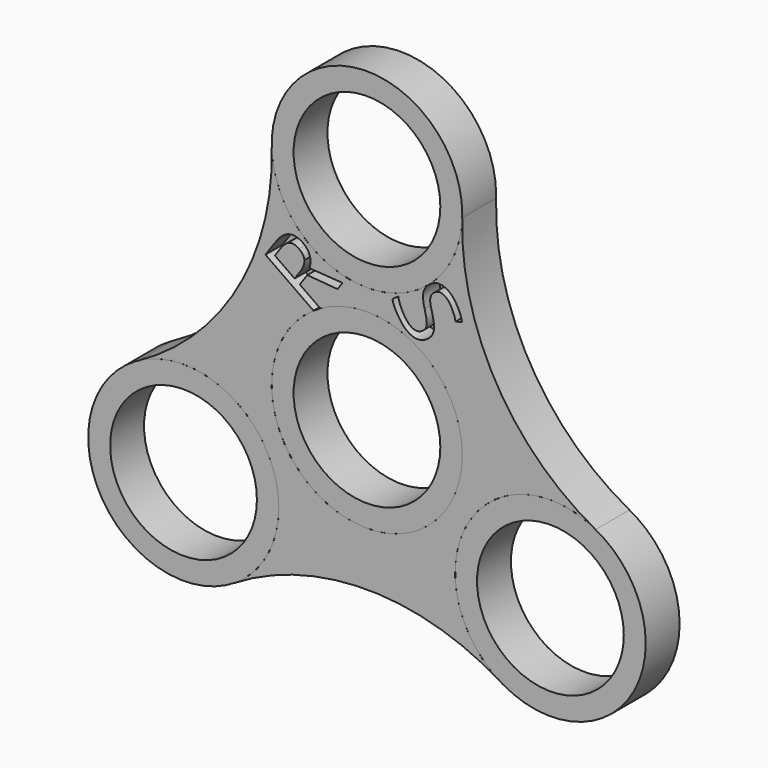
from build123d import *

# Parameters (mm, degrees)
F0_R         = 14.2875
F0_R_2       = 10.9982
F2_DEPTH     = 6.35
F1_R         = 14.2875
F3_TEXT_SIZE = 13.2291666667
F4_DEPTH     = 3.175


# Not quite as in the source:
# - Text() gives the source's letters only with a copy of the font that has no kerning and outlines rounded to 1/6400 em; it was checked with that copy


with BuildPart() as f2:
    # F0 (on Front) → F2 (new body)
    with BuildSketch(Plane.XZ):
        with Locations((0, 31.75)):
            Circle(F0_R)
        with Locations((0, 31.75)):
            Circle(F0_R_2, mode=Mode.SUBTRACT)
    extrude(amount=F2_DEPTH)


with BuildPart() as f2b:
    # F0 (on Front) → F2, piece 2 (new body)
    with BuildSketch(Plane.XZ):
        with Locations((-27.4963065702, -15.875)):
            Circle(F0_R)
        with Locations((-27.4963065702, -15.875)):
            Circle(F0_R_2, mode=Mode.SUBTRACT)
    extrude(amount=F2_DEPTH)


with BuildPart() as f2c:
    # F0 (on Front) → F2, piece 3 (new body)
    with BuildSketch(Plane.XZ):
        Circle(F0_R)
        Circle(F0_R_2, mode=Mode.SUBTRACT)
    extrude(amount=F2_DEPTH)


with BuildPart() as f2d:
    # F0 (on Front) → F2, piece 4 (new body)
    with BuildSketch(Plane.XZ):
        with Locations((27.4963065702, -15.875)):
            Circle(F0_R)
        with Locations((27.4963065702, -15.875)):
            Circle(F0_R_2, mode=Mode.SUBTRACT)
    extrude(amount=F2_DEPTH)


with BuildPart() as f2e:
    # F1 (on face) → F2, piece 5 (new body)
    with BuildSketch(Plane.XZ):
        with BuildLine():
            ThreePointArc((14.281510571, 31.3363430635), (0, 17.4625), (-14.281510571, 31.3363430635))
            ThreePointArc((-14.281510571, 31.3363430635), (-19.3699708761, 11.1832578995), (-34.2788244402, -3.3000205729))
            ThreePointArc((-34.2788244402, -3.3000205729), (-20.1741678054, -3.6063839346), (-13.2088065702, -15.875))
            ThreePointArc((-13.2088065702, -15.875), (-15.0208403571, -22.8388637995), (-19.9973138692, -28.0363224906))
            ThreePointArc((-19.9973138692, -28.0363224906), (0, -22.366515799), (19.9973138692, -28.0363224906))
            ThreePointArc((19.9973138692, -28.0363224906), (15.1229686136, -8.73125), (34.2788244402, -3.3000205729))
            ThreePointArc((34.2788244402, -3.3000205729), (19.3699708761, 11.1832578995), (14.281510571, 31.3363430635))
        make_face()
        Circle(F1_R, mode=Mode.SUBTRACT)
    extrude(amount=F2_DEPTH)

    # F3 (on face) → F4 (cut)
    with BuildSketch(Plane.XZ.offset(6.35)):
        with BuildLine():
            Line((-6.9997403161, 12.4553720039), (-10.0711094385, 14.605967816))
            Line((-10.0711094385, 14.605967816), (-8.9400323897, 16.2213132487))
            Line((-8.9400323897, 16.2213132487), (-4.4115968154, 15.841361106))
            Line((-4.4115968154, 15.841361106), (-3.6670303724, 16.9047121874))
            Line((-3.6670303724, 16.9047121874), (-8.6145888532, 17.2374768616))
            add(Edge.make_bspline(
                [(-9.5992202444, 20.245937907), (-8.0651500536, 19.1717703953), (-8.6145888532, 17.2374768616)],
                knots=[0, 0, 0, 1, 1, 1], degree=2))
            add(Edge.make_bspline(
                [(-11.7159887552, 20.7149656524), (-10.6947427758, 21.0130310418), (-9.5992202444, 20.245937907)],
                knots=[0, 0, 0, 1, 1, 1], degree=2))
            add(Edge.make_bspline(
                [(-13.7343372483, 18.9928902956), (-12.7372347346, 20.4169002629), (-11.7159887552, 20.7149656524)],
                knots=[0, 0, 0, 1, 1, 1], degree=2))
            Line((-13.7343372483, 18.9928902956), (-15.2199132882, 16.8712678353))
            Line((-15.2199132882, 16.8712678353), (-8.0159288261, 11.8269836098))
            ThreePointArc((-8.0159288261, 11.8269836098), (-7.5144060271, 12.1518047347), (-6.9997403161, 12.4553720039))
        make_face()
        with BuildLine():
            Line((-9.9789106426, 16.3809761542), (-10.8432242365, 15.1466084179))
            Line((-10.8432242365, 15.1466084179), (-13.8013043946, 17.2178784433))
            Line((-13.8013043946, 17.2178784433), (-12.9820441842, 18.3879032797))
            add(Edge.make_bspline(
                [(-11.6261393683, 19.6035751576), (-12.2813455094, 19.3886046955), (-12.9820441842, 18.3879032797)],
                knots=[0, 0, 0, 1, 1, 1], degree=2))
            add(Edge.make_bspline(
                [(-10.2038981319, 19.2814618637), (-10.9709332273, 19.8185456196), (-11.6261393683, 19.6035751576)],
                knots=[0, 0, 0, 1, 1, 1], degree=2))
            add(Edge.make_bspline(
                [(-9.3798086274, 18.042032789), (-9.4470224418, 18.7514918), (-10.2038981319, 19.2814618637)],
                knots=[0, 0, 0, 1, 1, 1], degree=2))
            add(Edge.make_bspline(
                [(-9.9789106426, 16.3809761542), (-9.3125948131, 17.3325737781), (-9.3798086274, 18.042032789)],
                knots=[0, 0, 0, 1, 1, 1], degree=2))
        make_face(mode=Mode.SUBTRACT)
        with Locations(Location((3.175, 17.607404383), (0, 0, -55))):
            Text('S', F3_TEXT_SIZE, font='Open Sans', text_align=(TextAlign.LEFT, TextAlign.BOTTOM))
    extrude(amount=-F4_DEPTH, mode=Mode.SUBTRACT)


solid = Compound([f2.part, f2b.part, f2c.part, f2d.part, f2e.part])
